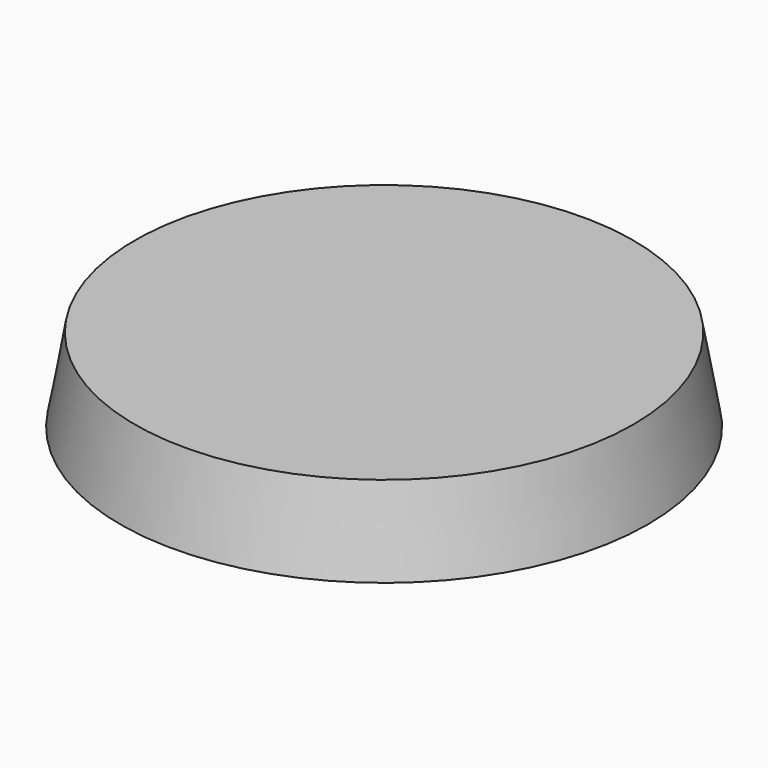
from build123d import *

# Parameters (mm, degrees)
F0_R         = 30
F1_DEPTH     = 10
F1_TAPER     = -10
F2_TEXT_SIZE = 20.8469055375
F3_DEPTH     = 1


# Not quite as in the source:
# - Text() gives the source's letters only with a copy of the font that has no kerning and outlines rounded to 1/6400 em; it was checked with that copy


with BuildPart() as f1:
    # F0 (on Top) → F1 (new body)
    with BuildSketch(Plane.XY):
        Circle(F0_R)
    extrude(amount=-F1_DEPTH, taper=F1_TAPER)

    # F2 (on face) → F3 (cut)
    with BuildSketch(Plane(origin=(0, 0, -10), x_dir=(1, 0, 0), z_dir=(0, 0, -1))):
        with Locations((-29, -5.009771987)):
            Text('Stefan', F2_TEXT_SIZE, font='Open Sans', font_style=FontStyle.ITALIC, text_align=(TextAlign.LEFT, TextAlign.BOTTOM))
    extrude(amount=-F3_DEPTH, mode=Mode.SUBTRACT)


solid = f1.part
